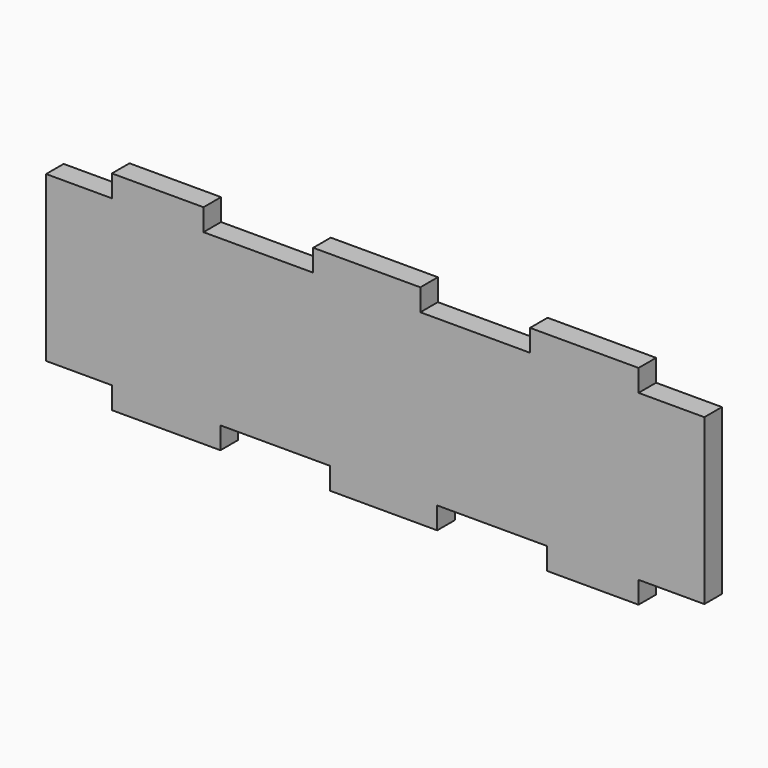
from build123d import *

# Parameters (mm, degrees)
F0_W     = 21.2041994
F0_H     = 5.08
F0_W_2   = 24.7952006
F0_W_3   = 25.1206
F0_W_4   = 24.7904
F0_W_5   = 21.209
F1_DEPTH = 5.08


# Not quite as in the source:
# - a feature names something its author has since deleted; it is built from what else it names


with BuildPart() as f1:
    # F0 (on Front) → F1 (new body)
    with BuildSketch(Plane.XZ):
        Polygon((60.96, -19.05), (76.2, -19.05), (76.2, 19.05), (60.96, 19.05), (35.8394, 19.05), (10.4394, 19.05), (-14.3558006, 19.05), (-39.7558006, 19.05), (-60.96, 19.05), (-76.2, 19.05), (-76.2, -19.05), (-60.96, -19.05), (-35.8394, -19.05), (-10.4394, -19.05), (14.351, -19.05), (39.751, -19.05), align=None)
        with Locations((-50.3579003, 21.59)):
            Rectangle(F0_W, F0_H)
        with Locations((-1.9582003, 21.59)):
            Rectangle(F0_W_2, F0_H)
        with Locations((48.3997, 21.59)):
            Rectangle(F0_W_3, F0_H)
        with Locations((1.9558, -21.59)):
            Rectangle(F0_W_4, F0_H)
        with Locations((50.3555, -21.59)):
            Rectangle(F0_W_5, F0_H)
        with Locations((-48.3997, -21.59)):
            Rectangle(F0_W_3, F0_H)
    extrude(amount=F1_DEPTH)


solid = f1.part
